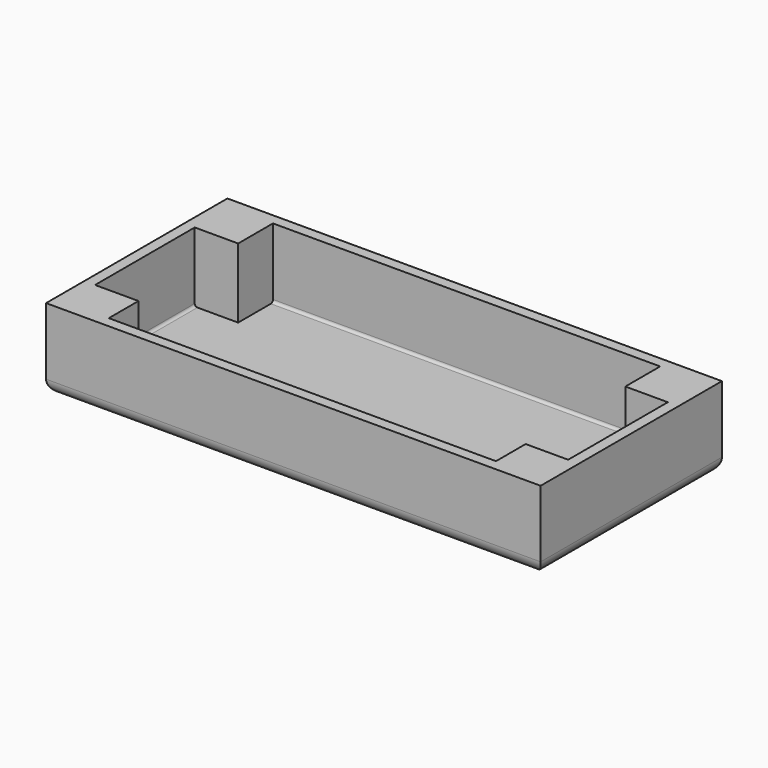
from build123d import *

# Parameters (mm, degrees)
F0_W     = 117.221
F0_H     = 53.721
F1_DEPTH = 19.05
F2_R     = 3.175
F3_T     = -2.54
F5_W     = 11.2527239306
F5_H     = 9.8262102796
F5_W_2   = 11.6953600091
F5_H_2   = 12.192
F6_DEPTH = 17.78


# Not quite as in the source:
# - a feature names something its author has since deleted; it is built from what else it names


with BuildPart() as f1:
    # F0 (on Top) → F1 (new body)
    with BuildSketch(Plane.XY):
        Rectangle(F0_W, F0_H)
    extrude(amount=F1_DEPTH)

    # F2
    f2_edges = [f1.edges().sort_by_distance(p)[0] for p in [
        (0, -26.8605, 0),
        (-58.6105, 0, 0),
        (0, 26.8605, 0),
        (58.6105, 0, 0),
    ]]
    fillet(f2_edges, radius=F2_R)

    # F3
    f3_openings = [f1.faces().sort_by_distance(p)[0] for p in [
        (0, 0, 19.05),
    ]]
    offset(amount=F3_T, openings=f3_openings)

    # F5 (on offset) → F6 (join)
    with BuildSketch(Plane.XY.offset(19.05)):
        with Locations((-51.4034552881, -20.4349435174)):
            Rectangle(F5_W, F5_H)
        with Locations((51.8481470752, 20.1015706725)):
            Rectangle(F5_W_2, F5_H_2)
        with Locations((-51.4034552881, 20.1015706725)):
            Rectangle(F5_W, F5_H_2)
        with Locations((51.8481470752, -20.4349435174)):
            Rectangle(F5_W_2, F5_H)
    extrude(amount=-F6_DEPTH)


solid = f1.part
